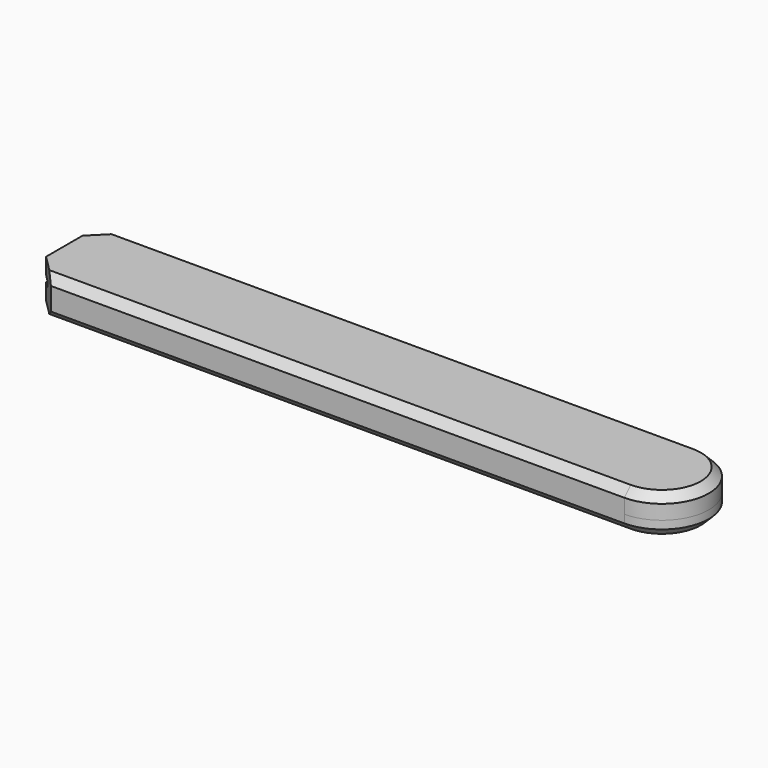
from build123d import *

# Parameters (mm, degrees)
F1_DEPTH    = 2
F2_DEPTH    = 0.8
F4_DEPTH    = 2
F5_SIZE     = 1
F6_T1_DEPTH = 18.2300979278


# Not quite as in the source:
# - a fillet or chamfer that OpenCascade refuses, or shapes differently, is made with other operations: its cross-section is extruded or revolved along the edge and cut away or added


with BuildPart() as f1:
    # F0 (on Top) → F1 (new body)
    with BuildSketch(Plane.XY):
        with BuildLine():
            Line((35.175, -3.825), (-39, -3.825))
            Line((-39, -3.825), (-39, -5.825))
            Line((-39, -5.825), (35.175, -5.825))
            ThreePointArc((35.175, -5.825), (39.2938970004, -4.1188970004), (41, 0))
            ThreePointArc((41, 0), (39.2938970004, 4.1188970004), (35.175, 5.825))
            Line((35.175, 5.825), (-39, 5.825))
            Line((-39, 5.825), (-39, 3.825))
            Line((-39, 3.825), (35.175, 3.825))
            ThreePointArc((35.175, 3.825), (37.879683438, 2.704683438), (39, 0))
            ThreePointArc((39, 0), (37.879683438, -2.704683438), (35.175, -3.825))
        make_face()
        with BuildLine():
            Line((-39, 3.825), (-39, -3.825))
            Line((-39, -3.825), (35.175, -3.825))
            ThreePointArc((35.175, -3.825), (37.879683438, -2.704683438), (39, 0))
            ThreePointArc((39, 0), (37.879683438, 2.704683438), (35.175, 3.825))
            Line((35.175, 3.825), (-39, 3.825))
        make_face()
    extrude(amount=F1_DEPTH)

    # F0 (on Top) → F2 (join)
    with BuildSketch(Plane.XY):
        with BuildLine():
            Line((35.175, -3.825), (-39, -3.825))
            Line((-39, -3.825), (-39, -5.825))
            Line((-39, -5.825), (35.175, -5.825))
            ThreePointArc((35.175, -5.825), (39.2938970004, -4.1188970004), (41, 0))
            ThreePointArc((41, 0), (39.2938970004, 4.1188970004), (35.175, 5.825))
            Line((35.175, 5.825), (-39, 5.825))
            Line((-39, 5.825), (-39, 3.825))
            Line((-39, 3.825), (35.175, 3.825))
            ThreePointArc((35.175, 3.825), (37.879683438, 2.704683438), (39, 0))
            ThreePointArc((39, 0), (37.879683438, -2.704683438), (35.175, -3.825))
        make_face()
    extrude(amount=-F2_DEPTH)

    # F3 (on face) → F4 (join)
    with BuildSketch(Plane(origin=(0, 0, -0.8), x_dir=(1, 0, 0), z_dir=(0, 0, -1))):
        with BuildLine():
            Line((-39, 3.825), (-39, -3.825))
            Line((-39, -3.825), (35.175, -3.825))
            ThreePointArc((35.175, -3.825), (39, 0), (35.175, 3.825))
            Line((35.175, 3.825), (-39, 3.825))
        make_face()
        with BuildLine():
            Line((35.175, -3.825), (-39, -3.825))
            Line((-39, -3.825), (-39, -5.825))
            Line((-39, -5.825), (35.175, -5.825))
            ThreePointArc((35.175, -5.825), (41, 0), (35.175, 5.825))
            Line((35.175, 5.825), (-39, 5.825))
            Line((-39, 5.825), (-39, 3.825))
            Line((-39, 3.825), (35.175, 3.825))
            ThreePointArc((35.175, 3.825), (39, 0), (35.175, -3.825))
        make_face()
    extrude(amount=F4_DEPTH)

    # F5
    f5_edges = [f1.edges().sort_by_distance(p)[0] for p in [
        (-1.9125, -5.825, -2.8),
        (-1.9125, -5.825, 2),
    ]]
    chamfer(f5_edges, length=F5_SIZE)

    # F6: chamfer of 3 on 2 edges, made by hand

    # F6_s2 → F6_t1 (cut)
    with BuildSketch(Plane.XY.offset(-9.5150489639)):
        Polygon((-39, -2.825), (-36, -5.825), (-39, -5.825), align=None)
        Polygon((-36, 5.825), (-39, 2.825), (-39, 5.825), align=None)
    extrude(amount=F6_T1_DEPTH, mode=Mode.SUBTRACT)


solid = f1.part
